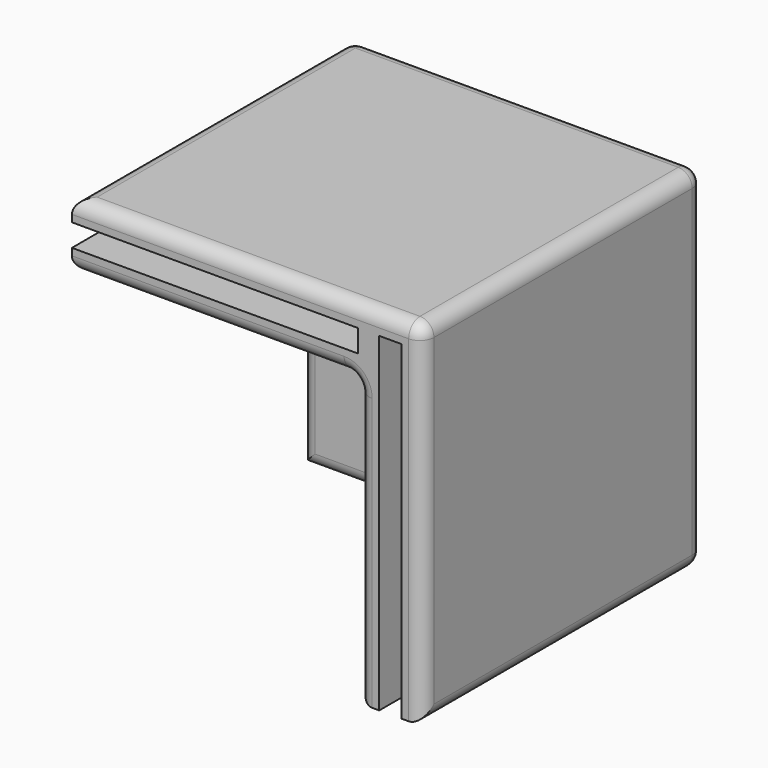
from build123d import *

# Parameters (mm, degrees)
F0_W      = 50
F0_H      = 50
F1_DEPTH  = 3
F2_W      = 3
F2_H      = 3
F2_H_2    = 47
F3_DEPTH  = 50
F4_W      = 3
F4_H      = 50
F5_DEPTH  = 47
F6_DEPTH  = 3
F7_W      = 3.2
F7_H      = 3.2
F8_DEPTH  = 50
F9_W      = 40.8
F9_H      = 3
F10_DEPTH = 40.8
F11_R     = 2


with BuildPart() as f1:
    # F0 (on Top) → F1 (new body)
    with BuildSketch(Plane.XY):
        Rectangle(F0_W, F0_H)
    extrude(amount=F1_DEPTH)

    # F2 (on face) → F3 (join, through all)
    with BuildSketch(Plane(origin=(-25, 0, 0), x_dir=(0, -1, 0), z_dir=(-1, 0, 0))):
        with Locations((-23.5, 1.5)):
            Rectangle(F2_W, F2_H)
        with Locations((-17.3, 1.5)):
            Rectangle(F2_W, F2_H)
        with Locations((-17.3, -23.5)):
            Rectangle(F2_W, F2_H_2)
        with Locations((-23.5, -23.5)):
            Rectangle(F2_W, F2_H_2)
    extrude(amount=-F3_DEPTH)

    # F4 (on face) → F5 (join, through all)
    with BuildSketch(Plane.XZ.offset(25)):
        with Locations((23.5, -22)):
            Rectangle(F4_W, F4_H)
        with Locations((17.3, -22)):
            Rectangle(F4_W, F4_H)
    extrude(amount=-F5_DEPTH)

    # F6 (add, through all): a face of the model
    f6_faces = [f1.faces().sort_by_distance(p)[0] for p in [
        (20.4, 20.4, 0),
    ]]
    extrude(f6_faces, amount=-F6_DEPTH)

    # F7 (on face) → F8 (join, through all)
    with BuildSketch(Plane(origin=(0, 0, -47), x_dir=(1, 0, 0), z_dir=(0, 0, -1))):
        with Locations((20.4, -20.4)):
            Rectangle(F7_W, F7_H)
    extrude(amount=-F8_DEPTH)

    # F9 (on face) → F10 (join, through all)
    with BuildSketch(Plane(origin=(-25, 0, 0), x_dir=(0, -1, 0), z_dir=(-1, 0, 0))):
        with Locations((4.6, -4.7)):
            Rectangle(F9_W, F9_H)
    extrude(amount=-F10_DEPTH)

    # F11
    f11_edges = [f1.edges().sort_by_distance(p)[0] for p in [
        (-25, 0, 3),
        (0, -25, 3),
        (0, 25, 3),
        (25, 0, 3),
        (25, 0, -47),
        (25, -25, -22),
        (25, 25, -22),
        (-25, 25, -22),
        (0, 25, -47),
        (15.8, -25, -26.6),
        (15.8, -4.6, -47),
        (15.8, 15.8, -26.6),
        (15.8, -4.6, -6.2),
        (-25, 15.8, -26.6),
        (-4.6, 15.8, -6.2),
        (-4.6, 15.8, -47),
        (-4.6, -25, -6.2),
        (-25, -4.6, -6.2),
    ]]
    fillet(f11_edges, radius=F11_R)


solid = f1.part
